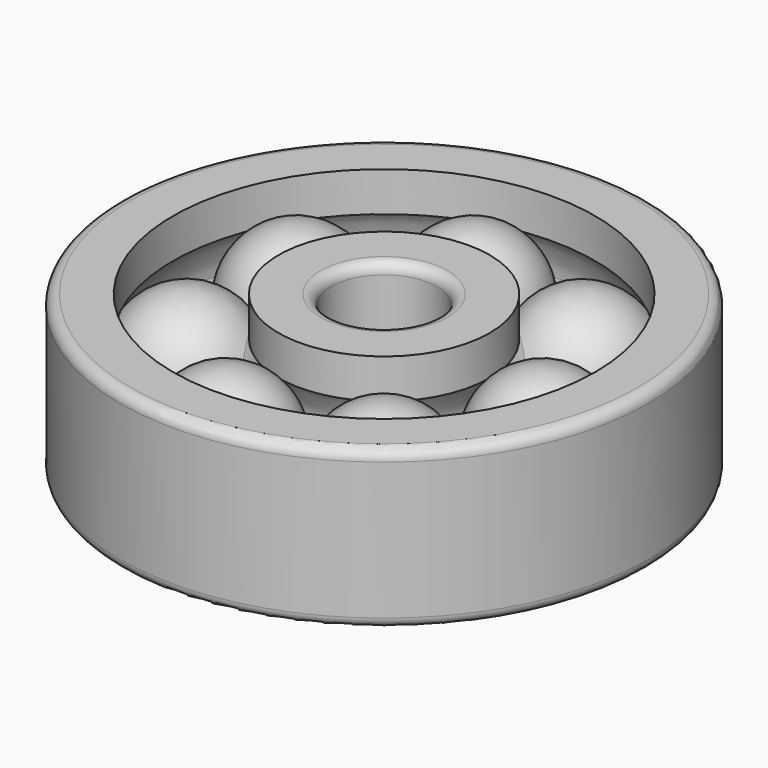
from build123d import *

# Parameters (mm, degrees)
F3_COUNT = 7
F4_R     = 2.54
F4_2_R   = 2.54


# Not quite as in the source:
# - after a boolean that leaves OpenCascade's solid faulty, fix() repairs it


with BuildPart() as f1:
    # F0 (on Front) → F1 (revolve)
    with BuildSketch(Plane.XZ):
        with BuildLine():
            Line((25.4, 19.05), (12.7, 19.05))
            Line((12.7, 19.05), (12.7, -19.05))
            Line((12.7, -19.05), (25.4, -19.05))
            Line((25.4, -19.05), (25.4, -9.525))
            ThreePointArc((25.4, -9.525), (23.0396526434, -5.0201157855), (22.225, 0))
            ThreePointArc((22.225, 0), (23.0396526434, 5.0201157855), (25.4, 9.525))
            Line((25.4, 9.525), (25.4, 19.05))
        make_face()
    revolve(axis=Axis((0, 0, 0), (0, 0, -1)))

    # F4#2
    f4_2_edges = [f1.edges().sort_by_distance(p)[0] for p in [
        (-12.7, 0, -19.05),
        (-12.7, 0, 19.05),
    ]]
    fillet(f4_2_edges, radius=F4_2_R)


with BuildPart() as f1b:
    # F0 (on Front) → F1, piece 2 (revolve)
    with BuildSketch(Plane.XZ):
        with BuildLine():
            Line((50.8, 19.05), (50.8, 9.525))
            ThreePointArc((50.8, 9.525), (53.1603473566, 5.0201157855), (53.975, 0))
            ThreePointArc((53.975, 0), (53.1603473566, -5.0201157855), (50.8, -9.525))
            Line((50.8, -9.525), (50.8, -19.05))
            Line((50.8, -19.05), (63.5, -19.05))
            Line((63.5, -19.05), (63.5, 19.05))
            Line((63.5, 19.05), (50.8, 19.05))
        make_face()
    revolve(axis=Axis((0, 0, 0), (0, 0, -1)))

    # F4
    f4_edges = [f1b.edges().sort_by_distance(p)[0] for p in [
        (-63.5, 0, 19.05),
        (-63.5, 0, -19.05),
    ]]
    fillet(f4_edges, radius=F4_R)


with BuildPart() as f2:
    # F0 (on Front) → F2 (revolve)
    with BuildSketch(Plane.XZ):
        with BuildLine():
            Line((25.4, 0), (25.4, 9.525))
            ThreePointArc((25.4, 9.525), (23.0396526434, 5.0201157855), (22.225, 0))
            Line((22.225, 0), (25.4, 0))
        make_face()
        with BuildLine():
            ThreePointArc((50.8, 9.525), (38.1, 15.875), (25.4, 9.525))
            Line((25.4, 9.525), (25.4, 0))
            Line((25.4, 0), (50.8, 0))
            Line((50.8, 0), (50.8, 9.525))
        make_face()
        with BuildLine():
            Line((50.8, 0), (50.8, -9.525))
            ThreePointArc((50.8, -9.525), (53.1603473566, -5.0201157855), (53.975, 0))
            Line((53.975, 0), (50.8, 0))
        make_face()
    revolve(axis=Axis((38.1, 0, 0), (1, 0, 0)))

    add(f2.part.fix(), mode=Mode.REPLACE)


with BuildPart() as f3_1:
    # F3: instance of F2
    add(f2.part.rotate(Axis((0, 0, 0), (0, 0, -1)), 1 * 360 / F3_COUNT))


with BuildPart() as f3_2:
    # F3: instance of F2
    add(f2.part.rotate(Axis((0, 0, 0), (0, 0, -1)), 2 * 360 / F3_COUNT))


with BuildPart() as f3_3:
    # F3: instance of F2
    add(f2.part.rotate(Axis((0, 0, 0), (0, 0, -1)), 3 * 360 / F3_COUNT))


with BuildPart() as f3_4:
    # F3: instance of F2
    add(f2.part.rotate(Axis((0, 0, 0), (0, 0, -1)), 4 * 360 / F3_COUNT))


with BuildPart() as f3_5:
    # F3: instance of F2
    add(f2.part.rotate(Axis((0, 0, 0), (0, 0, -1)), 5 * 360 / F3_COUNT))


with BuildPart() as f3_6:
    # F3: instance of F2
    add(f2.part.rotate(Axis((0, 0, 0), (0, 0, -1)), 6 * 360 / F3_COUNT))


solid = Compound([f1.part, f1b.part, f2.part, f3_1.part, f3_2.part, f3_3.part, f3_4.part, f3_5.part, f3_6.part])
